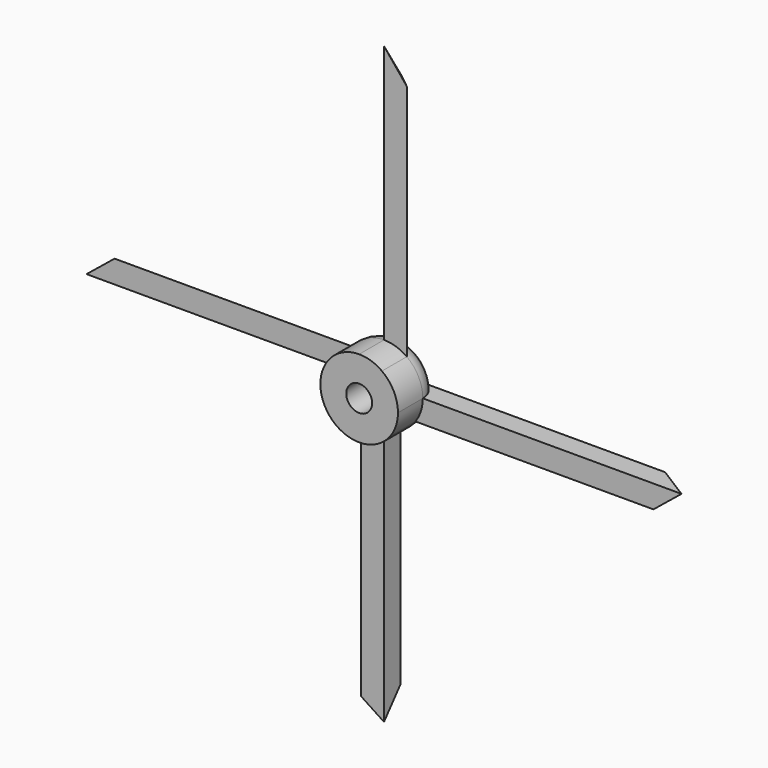
from build123d import *

# Parameters (mm, degrees)
F0_R         = 3.175
F1_DEPTH     = 12.7
F2_DEPTH     = 5.08
F3_SIZE      = 5.07999
F4_T3_ANGLE  = 206.8900819295
F4_T7_ANGLE  = 130.484631046
F4_T11_ANGLE = 206.8900819295
F4_T15_ANGLE = 206.8900819295
F4_T19_ANGLE = 130.484631046
F4_T23_ANGLE = 206.8900819295
F4_T27_ANGLE = 206.8900819295
F4_T31_ANGLE = 130.484631046
F4_T35_ANGLE = 206.8900819295
F4_T39_ANGLE = 206.8900819295
F4_T43_ANGLE = 130.484631046
F4_T47_ANGLE = 206.8900819295


# Not quite as in the source:
# - a fillet or chamfer that OpenCascade refuses, or shapes differently, is made with other operations: its cross-section is extruded or revolved along the edge and cut away or added
# - a fillet or chamfer is up to 0.001 mm smaller than in the source, because OpenCascade refuses the exact size


with BuildPart() as f1:
    # F0 (on Front) → F1 (new body)
    with BuildSketch(Plane.XZ):
        with BuildLine():
            ThreePointArc((15.8353851332, 8.5368495443), (17.1826135049, 11.1877228091), (17.6467685365, 14.1248495443))
            ThreePointArc((17.6467685365, 14.1248495443), (16.6056156886, 18.4549722331), (13.7097685365, 21.838466141))
            ThreePointArc((13.7097685365, 21.838466141), (11.0588952717, 23.1856945127), (8.1217685365, 23.6498495443))
            ThreePointArc((8.1217685365, 23.6498495443), (3.7916458477, 22.6086966964), (0.4081519399, 19.7128495443))
            ThreePointArc((0.4081519399, 19.7128495443), (-0.9390764319, 17.0619762795), (-1.4032314635, 14.1248495443))
            ThreePointArc((-1.4032314635, 14.1248495443), (-0.3620786156, 9.7947268555), (2.5337685365, 6.4112329477))
            ThreePointArc((2.5337685365, 6.4112329477), (5.1846418013, 5.0640045759), (8.1217685365, 4.5998495443))
            ThreePointArc((8.1217685365, 4.5998495443), (12.4518912253, 5.6410023922), (15.8353851332, 8.5368495443))
        make_face()
        with Locations((8.1217685365, 14.1248495443)):
            Circle(F0_R, mode=Mode.SUBTRACT)
    extrude(amount=F1_DEPTH)

    # F0 (on Front) → F2 (join)
    with BuildSketch(Plane.XZ):
        with BuildLine():
            ThreePointArc((8.1217685365, 23.6498495443), (11.0588952717, 23.1856945127), (13.7097685365, 21.838466141))
            Line((13.7097685365, 21.838466141), (13.7097685365, 80.258466141))
            Line((13.7097685365, 80.258466141), (8.1217685365, 87.1498495443))
            Line((8.1217685365, 87.1498495443), (8.1217685365, 23.6498495443))
        make_face()
        with BuildLine():
            Line((81.1467685365, 14.1248495443), (17.6467685365, 14.1248495443))
            ThreePointArc((17.6467685365, 14.1248495443), (17.1826135049, 11.1877228091), (15.8353851332, 8.5368495443))
            Line((15.8353851332, 8.5368495443), (74.2553851332, 8.5368495443))
            Line((74.2553851332, 8.5368495443), (81.1467685365, 14.1248495443))
        make_face()
        with BuildLine():
            ThreePointArc((-1.4032314635, 14.1248495443), (-0.9390764319, 17.0619762795), (0.4081519399, 19.7128495443))
            Line((0.4081519399, 19.7128495443), (-58.0118480601, 19.7128495443))
            Line((-58.0118480601, 19.7128495443), (-64.9032314635, 14.1248495443))
            Line((-64.9032314635, 14.1248495443), (-1.4032314635, 14.1248495443))
        make_face()
        with BuildLine():
            Line((8.1217685365, -58.9001504557), (8.1217685365, 4.5998495443))
            ThreePointArc((8.1217685365, 4.5998495443), (5.1846418013, 5.0640045759), (2.5337685365, 6.4112329477))
            Line((2.5337685365, 6.4112329477), (2.5337685365, -55.2206523716))
            Line((2.5337685365, -55.2206523716), (8.1217685365, -58.9001504557))
        make_face()
    extrude(amount=F2_DEPTH)

    # F3 (size 5.08 in the source; OpenCascade refuses exactly that, so slightly less here)
    f3_edges = [f1.edges().sort_by_distance(p)[0] for p in [
        (77.701077, 0, 11.33085),
        (45.045385, 0, 8.53685),
        (13.709769, 0, 51.048466),
        (10.915769, 0, 83.704158),
        (2.533769, 0, -24.40471),
        (5.327769, 0, -57.060401),
        (-28.801848, 0, 19.71285),
        (-61.45754, 0, 16.91885),
    ]]
    chamfer(f3_edges, length=F3_SIZE)

    # F4: fillet of radius 5.08 on 4 edges, made by hand


with BuildPart() as f4_tool1:
    # F4_s2 → F4_t3 (revolve)
    with BuildSketch(Plane(origin=(10.9000788328, 0, 2.6359089402), x_dir=(0, 1, 0), z_dir=(-0.9719833666, 0, -0.2350496437))):
        with BuildLine():
            ThreePointArc((-5.08, -2.2951000126), (-1.4878975516, -3.7829975641), (0, -7.3751000126))
            Line((0, -7.3751000126), (0, -2.2951000126))
            Line((0, -2.2951000126), (-5.08, -2.2951000126))
        make_face()
    revolve(axis=Axis((8.1217685365, 0, 14.1248495443), (0, -1, 0)), revolution_arc=F4_T3_ANGLE)

    split(bisect_by=Plane(origin=(0, -6.8084197722, 6.8084197722), x_dir=(1, 0, 0), z_dir=(0, 0.7071067812, -0.7071067812)), keep=Keep.TOP)


with BuildPart() as f4_tool5:
    # F4_s6 → F4_t7 (revolve)
    with BuildSketch(Plane.XY.offset(14.1248495443)):
        with BuildLine():
            ThreePointArc((17.6467685365, -5.08), (16.158870985, -1.4878975516), (12.5667685365, 0))
            Line((12.5667685365, 0), (17.6467685365, 0))
            Line((17.6467685365, 0), (17.6467685365, -5.08))
        make_face()
    revolve(axis=Axis((8.1217685365, 0, 14.1248495443), (0, -1, 0)), revolution_arc=F4_T7_ANGLE)

    split(bisect_by=Plane(origin=(4.3148892683, 4.3148892683, 0), x_dir=(0, 0, 1), z_dir=(0.7071067812, 0.7071067812, 0)), keep=Keep.TOP)


with BuildPart() as f4_tool9:
    # F4_s10 → F4_t11 (revolve)
    with BuildSketch(Plane(origin=(10.9000788328, 0, 2.6359089402), x_dir=(0, 1, 0), z_dir=(-0.9719833666, 0, -0.2350496437))):
        with BuildLine():
            ThreePointArc((-5.08, -2.2951000126), (-1.4878975516, -3.7829975641), (0, -7.3751000126))
            Line((0, -7.3751000126), (0, -2.2951000126))
            Line((0, -2.2951000126), (-5.08, -2.2951000126))
        make_face()
    revolve(axis=Axis((8.1217685365, 0, 14.1248495443), (0, -1, 0)), revolution_arc=F4_T11_ANGLE)

    split(bisect_by=Plane.YZ.offset(8.1217685365), keep=Keep.BOTTOM)


with BuildPart() as f4_tool13:
    # F4_s14 → F4_t15 (revolve)
    with BuildSketch(Plane(origin=(-2.7783102963, 0, 11.4889406041), x_dir=(0, 1, 0), z_dir=(-0.2350496437, 0, 0.9719833666))):
        with BuildLine():
            ThreePointArc((-5.08, -1.6892647777), (-1.4878975516, -3.1771623292), (0, -6.7692647777))
            Line((0, -6.7692647777), (0, -1.6892647777))
            Line((0, -1.6892647777), (-5.08, -1.6892647777))
        make_face()
    revolve(axis=Axis((8.1217685365, 0, 14.1248495443), (0, -1, 0)), revolution_arc=F4_T15_ANGLE)

    split(bisect_by=Plane(origin=(3.8068792683, -3.8068792683, 0), x_dir=(0, 0, 1), z_dir=(-0.7071067812, 0.7071067812, 0)), keep=Keep.TOP)


with BuildPart() as f4_tool17:
    # F4_s18 → F4_t19 (revolve)
    with BuildSketch(Plane.YZ.offset(8.1217685365)):
        with BuildLine():
            ThreePointArc((-5.08, 4.5998495443), (-1.4878975516, 6.0877470959), (0, 9.6798495443))
            Line((0, 9.6798495443), (0, 4.5998495443))
            Line((0, 4.5998495443), (-5.08, 4.5998495443))
        make_face()
    revolve(axis=Axis((8.1217685365, 0, 14.1248495443), (0, -1, 0)), revolution_arc=F4_T19_ANGLE)

    split(bisect_by=Plane(origin=(0, -6.8084197722, 6.8084197722), x_dir=(1, 0, 0), z_dir=(0, 0.7071067812, -0.7071067812)), keep=Keep.TOP)


with BuildPart() as f4_tool21:
    # F4_s22 → F4_t23 (revolve)
    with BuildSketch(Plane(origin=(-2.7783102963, 0, 11.4889406041), x_dir=(0, 1, 0), z_dir=(-0.2350496437, 0, 0.9719833666))):
        with BuildLine():
            ThreePointArc((-5.08, -1.6892647777), (-1.4878975516, -3.1771623292), (0, -6.7692647777))
            Line((0, -6.7692647777), (0, -1.6892647777))
            Line((0, -1.6892647777), (-5.08, -1.6892647777))
        make_face()
    revolve(axis=Axis((8.1217685365, 0, 14.1248495443), (0, -1, 0)), revolution_arc=F4_T23_ANGLE)

    split(bisect_by=Plane.XY.offset(14.1248495443), keep=Keep.TOP)


with BuildPart() as f4_tool25:
    # F4_s26 → F4_t27 (revolve)
    with BuildSketch(Plane(origin=(-2.7783102963, 0, 11.4889406041), x_dir=(0, 1, 0), z_dir=(0.2350496437, 0, -0.9719833666))):
        with BuildLine():
            ThreePointArc((-5.08, 20.7392647777), (-1.4878975516, 19.2513672261), (0, 15.6592647777))
            Line((0, 15.6592647777), (0, 20.7392647777))
            Line((0, 20.7392647777), (-5.08, 20.7392647777))
        make_face()
    revolve(axis=Axis((8.1217685365, 0, 14.1248495443), (0, -1, 0)), revolution_arc=F4_T27_ANGLE)

    split(bisect_by=Plane(origin=(4.3148892683, 4.3148892683, 0), x_dir=(0, 0, 1), z_dir=(0.7071067812, 0.7071067812, 0)), keep=Keep.TOP)


with BuildPart() as f4_tool29:
    # F4_s30 → F4_t31 (revolve)
    with BuildSketch(Plane.YZ.offset(8.1217685365)):
        with BuildLine():
            ThreePointArc((-5.08, 23.6498495443), (-1.4878975516, 22.1619519927), (0, 18.5698495443))
            Line((0, 18.5698495443), (0, 23.6498495443))
            Line((0, 23.6498495443), (-5.08, 23.6498495443))
        make_face()
    revolve(axis=Axis((8.1217685365, 0, 14.1248495443), (0, -1, 0)), revolution_arc=F4_T31_ANGLE)

    split(bisect_by=Plane(origin=(0, 7.3164297722, 7.3164297722), x_dir=(1, 0, 0), z_dir=(0, 0.7071067812, 0.7071067812)), keep=Keep.TOP)


with BuildPart() as f4_tool33:
    # F4_s34 → F4_t35 (revolve)
    with BuildSketch(Plane(origin=(-2.7783102963, 0, 11.4889406041), x_dir=(0, 1, 0), z_dir=(0.2350496437, 0, -0.9719833666))):
        with BuildLine():
            ThreePointArc((-5.08, 20.7392647777), (-1.4878975516, 19.2513672261), (0, 15.6592647777))
            Line((0, 15.6592647777), (0, 20.7392647777))
            Line((0, 20.7392647777), (-5.08, 20.7392647777))
        make_face()
    revolve(axis=Axis((8.1217685365, 0, 14.1248495443), (0, -1, 0)), revolution_arc=F4_T35_ANGLE)

    split(bisect_by=Plane.XY.offset(14.1248495443), keep=Keep.BOTTOM)


with BuildPart() as f4_tool37:
    # F4_s38 → F4_t39 (revolve)
    with BuildSketch(Plane(origin=(10.9000788328, 0, 2.6359089402), x_dir=(0, 1, 0), z_dir=(0.9719833666, 0, 0.2350496437))):
        with BuildLine():
            ThreePointArc((-5.08, 21.3451000126), (-1.4878975516, 19.857202461), (0, 16.2651000126))
            Line((0, 16.2651000126), (0, 21.3451000126))
            Line((0, 21.3451000126), (-5.08, 21.3451000126))
        make_face()
    revolve(axis=Axis((8.1217685365, 0, 14.1248495443), (0, -1, 0)), revolution_arc=F4_T39_ANGLE)

    split(bisect_by=Plane(origin=(0, 7.3164297722, 7.3164297722), x_dir=(1, 0, 0), z_dir=(0, 0.7071067812, 0.7071067812)), keep=Keep.TOP)


with BuildPart() as f4_tool41:
    # F4_s42 → F4_t43 (revolve)
    with BuildSketch(Plane.XY.offset(14.1248495443)):
        with BuildLine():
            ThreePointArc((-1.4032314635, -5.08), (0.0846660881, -1.4878975516), (3.6767685365, 0))
            Line((3.6767685365, 0), (-1.4032314635, 0))
            Line((-1.4032314635, 0), (-1.4032314635, -5.08))
        make_face()
    revolve(axis=Axis((8.1217685365, 0, 14.1248495443), (0, -1, 0)), revolution_arc=F4_T43_ANGLE)

    split(bisect_by=Plane(origin=(3.8068792683, -3.8068792683, 0), x_dir=(0, 0, 1), z_dir=(-0.7071067812, 0.7071067812, 0)), keep=Keep.TOP)


with BuildPart() as f4_tool45:
    # F4_s46 → F4_t47 (revolve)
    with BuildSketch(Plane(origin=(10.9000788328, 0, 2.6359089402), x_dir=(0, 1, 0), z_dir=(0.9719833666, 0, 0.2350496437))):
        with BuildLine():
            ThreePointArc((-5.08, 21.3451000126), (-1.4878975516, 19.857202461), (0, 16.2651000126))
            Line((0, 16.2651000126), (0, 21.3451000126))
            Line((0, 21.3451000126), (-5.08, 21.3451000126))
        make_face()
    revolve(axis=Axis((8.1217685365, 0, 14.1248495443), (0, -1, 0)), revolution_arc=F4_T47_ANGLE)

    split(bisect_by=Plane.YZ.offset(8.1217685365), keep=Keep.TOP)


with BuildPart() as f1_1:
    add(f1.part)

    # F4_t49: cut F4_tool1, F4_tool5, F4_tool9, F4_tool13, F4_tool17, F4_tool21, F4_tool25, F4_tool29, F4_tool33, F4_tool37, F4_tool41, F4_tool45
    add([f4_tool1.part, f4_tool5.part, f4_tool9.part, f4_tool13.part, f4_tool17.part, f4_tool21.part, f4_tool25.part, f4_tool29.part, f4_tool33.part, f4_tool37.part, f4_tool41.part, f4_tool45.part], mode=Mode.SUBTRACT)


solid = f1_1.part
